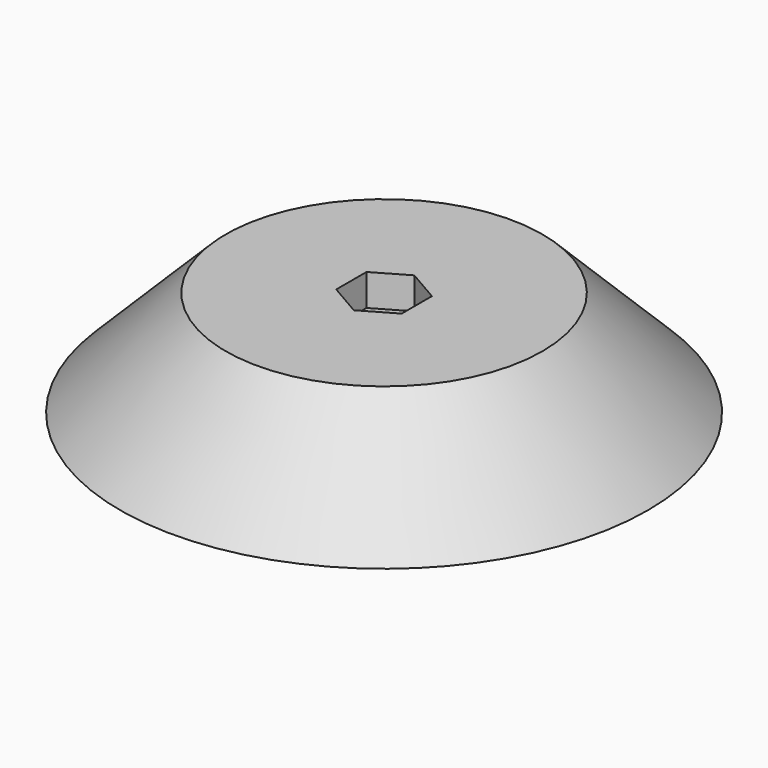
from build123d import *

# Parameters (mm, degrees)
F2_R     = 25.4
F2_R_2   = 1.7145
F4_DEPTH = 12.7
F0_R     = 31.75
F0_R_2   = 1.7145
F5_DEPTH = 12.7
F6_R     = 1.7145
F7_DEPTH = 3.81
F8_SIZE2 = 12.69999
F8_SIZE  = 12.69999


# Not quite as in the source:
# - a fillet or chamfer is up to 0.001 mm smaller than in the source, because OpenCascade refuses the exact size


with BuildPart() as f4:
    # F2 (on offset) → F4 (new body)
    with BuildSketch(Plane.XY.offset(12.7)):
        with Locations((-31.75, 31.75)):
            Circle(F2_R)
        with Locations((-31.75, 31.75)):
            Circle(F2_R_2, mode=Mode.SUBTRACT)
    extrude(amount=-F4_DEPTH)

    # F0 (on Top) → F5 (join)
    with BuildSketch(Plane.XY):
        with Locations((-31.75, 31.75)):
            Circle(F0_R)
        with Locations((-31.75, 31.75)):
            Circle(F0_R_2, mode=Mode.SUBTRACT)
    extrude(amount=F5_DEPTH)

    # F6 (on face) → F7 (cut)
    with BuildSketch(Plane.XY.offset(12.7)):
        Polygon((-27.813, 29.4769719902), (-27.813, 34.0230280098), (-31.75, 36.2960560196), (-35.687, 34.0230280098), (-35.687, 29.4769719902), (-31.75, 27.2039439804), align=None)
        with Locations((-31.75, 31.75)):
            Circle(F6_R, mode=Mode.SUBTRACT)
    extrude(amount=-F7_DEPTH, mode=Mode.SUBTRACT)

    # F8 (size 12.7 and 12.7 in the source; OpenCascade refuses exactly that, so slightly less here)
    f8_edges = [f4.edges().sort_by_distance(p)[0] for p in [
        (-63.5, 31.75, 12.7),
    ]]
    chamfer(f8_edges, length=F8_SIZE, length2=F8_SIZE2)


solid = f4.part
